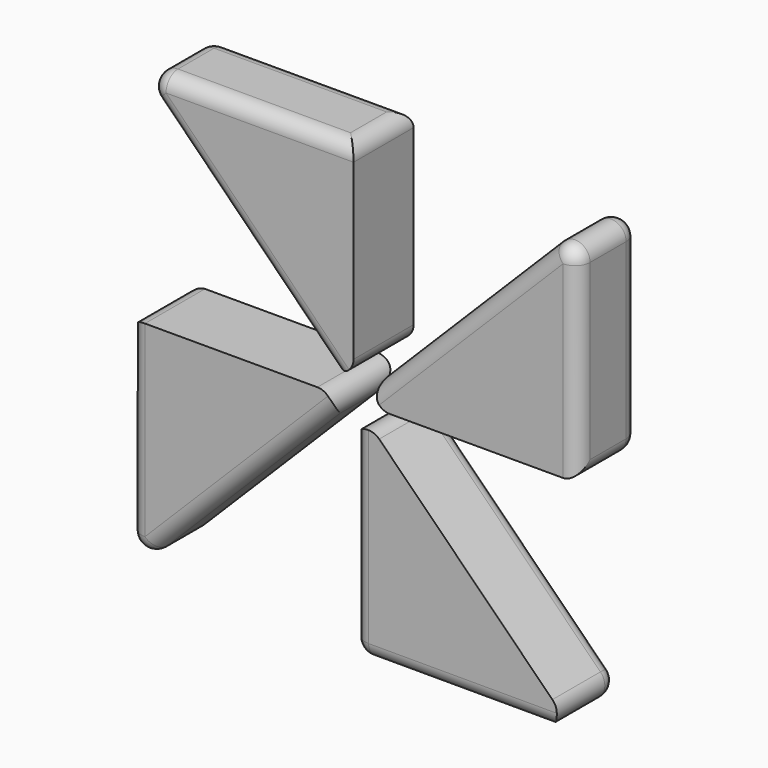
from build123d import *

# Parameters (mm, degrees)
F1_DEPTH = 25.4
F2_R     = 5.08
F2_2_R   = 5.08
F2_3_R   = 5.08
F2_4_R   = 5.08


with BuildPart() as f1:
    # F0 (on Front) → F1 (new body)
    with BuildSketch(Plane.XZ):
        Polygon((76.0156884789, -75.9169031134), (0, 0), (0, -75.8305569174), align=None)
    extrude(amount=F1_DEPTH)

    # F2
    f2_edges = [f1.edges().sort_by_distance(p)[0] for p in [
        (0, -12.7, -75.830557),
        (76.015688, -12.7, -75.916903),
        (38.007844, 0, -75.87373),
        (38.007844, -25.4, -75.87373),
        (0, 0, -37.915278),
        (0, -25.4, -37.915278),
        (38.007844, 0, -37.958452),
        (0, -12.7, 0),
    ]]
    fillet(f2_edges, radius=F2_R)


with BuildPart() as f1b:
    # F0 (on Front) → F1, piece 2 (new body)
    with BuildSketch(Plane.XZ):
        Polygon((-75.714327395, 76.114602387), (0, 0), (0, 76.114602387), align=None)
    extrude(amount=F1_DEPTH)

    # F2#2
    f2_2_edges = [f1b.edges().sort_by_distance(p)[0] for p in [
        (-75.714327, -12.7, 76.114602),
        (-37.857164, 0, 38.057301),
        (-37.857164, -25.4, 38.057301),
        (0, -12.7, 76.114602),
        (-37.857164, 0, 76.114602),
        (-37.857164, -25.4, 76.114602),
        (0, -12.7, 0),
    ]]
    fillet(f2_2_edges, radius=F2_2_R)


with BuildPart() as f1c:
    # F0 (on Front) → F1, piece 3 (new body)
    with BuildSketch(Plane.XZ):
        Polygon((76.0156884789, 76.114602387), (0, 0), (76.0156884789, 0), align=None)
    extrude(amount=F1_DEPTH)

    # F2#3
    f2_3_edges = [f1c.edges().sort_by_distance(p)[0] for p in [
        (76.015688, -12.7, 0),
        (76.015688, -12.7, 76.114602),
        (76.015688, 0, 38.057301),
        (76.015688, -25.4, 38.057301),
        (38.007844, 0, 0),
        (0, -12.7, 0),
        (38.007844, 0, 38.057301),
        (38.007844, -25.4, 38.057301),
    ]]
    fillet(f2_3_edges, radius=F2_3_R)


with BuildPart() as f1d:
    # F0 (on Front) → F1, piece 4 (new body)
    with BuildSketch(Plane.XZ):
        Polygon((-75.7320121376, -75.8305569174), (0, 0), (-75.714327395, 0), align=None)
    extrude(amount=F1_DEPTH)

    # F2#4
    f2_4_edges = [f1d.edges().sort_by_distance(p)[0] for p in [
        (0, -12.7, 0),
        (-75.732012, -12.7, -75.830557),
        (-37.866006, 0, -37.915278),
        (-37.866006, -25.4, -37.915278),
        (-75.714327, -12.7, 0),
        (-75.72317, 0, -37.915278),
        (-75.72317, -25.4, -37.915278),
    ]]
    fillet(f2_4_edges, radius=F2_4_R)


solid = Compound([f1.part, f1b.part, f1c.part, f1d.part])
